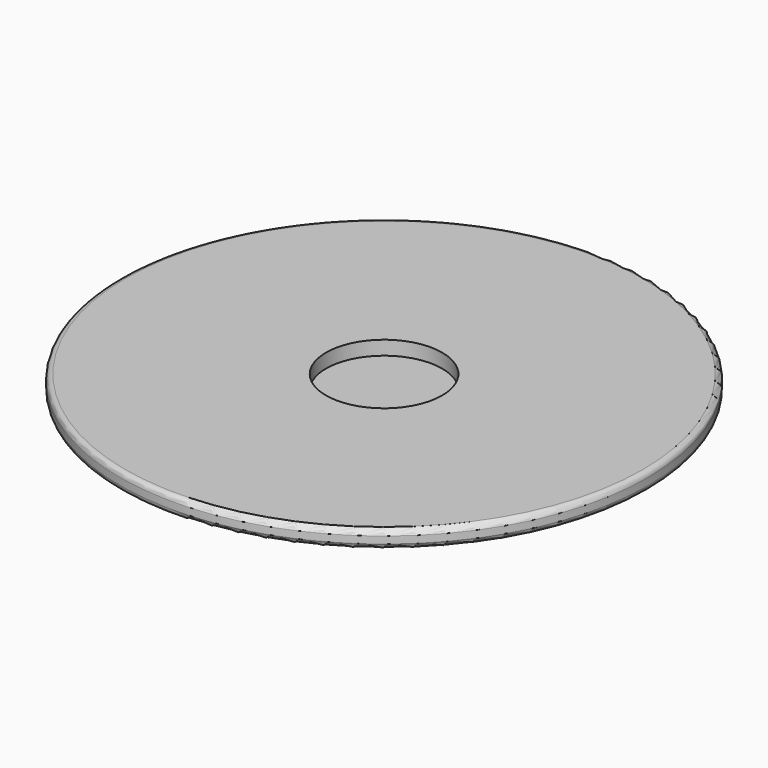
from build123d import *

# Parameters (mm, degrees)
F0_R     = 7.5
F1_DEPTH = 0.5
F2_R     = 0.15
F3_R     = 1.65
F4_DEPTH = 0.4


# Not quite as in the source:
# - a feature names something its author has since deleted; it is built from what else it names


with BuildPart() as f1:
    # F0 (on Top) → F1 (new body)
    with BuildSketch(Plane.XY):
        Circle(F0_R)
    extrude(amount=F1_DEPTH)

    # F2
    f2_edges = [f1.edges().sort_by_distance(p)[0] for p in [
        (-7.5, 0, 0.5),
        (-7.5, 0, 0),
    ]]
    fillet(f2_edges, radius=F2_R)

    # F3 (on face) → F4 (cut)
    with BuildSketch(Plane.XY.offset(0.5)):
        Circle(F3_R)
    extrude(amount=-F4_DEPTH, mode=Mode.SUBTRACT)


solid = f1.part
